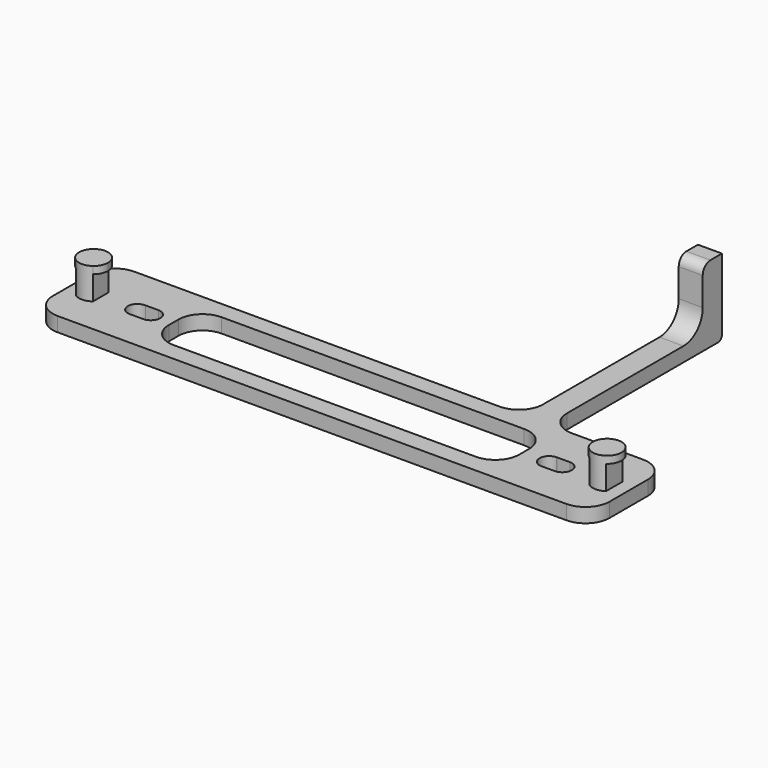
from build123d import *

# Parameters (mm, degrees)
F0_W     = 5
F0_H     = 40.3502766341
F0_H_2   = 5
F0_H_3   = 3.6678295396
F1_DEPTH = 3
F2_DEPTH = 8
F3_START = 8
F3_DEPTH = 1.5
F4_DEPTH = 15.9
F5_R     = 5
F6_R     = 2
F7_R     = 5
F8_R     = 5
F9_R     = 1


# Not quite as in the source:
# - a feature names something its author has since deleted; it is built from what else it names


with BuildPart() as f1:
    # F0 (on Top) → F1 (new body)
    with BuildSketch(Plane.XY):
        Polygon((28.0917086639, 10.1497233659), (-58.0486447513, 10.1497233659), (-58.0486447513, -9.8502766341), (57.9513552487, -9.8502766341), (57.9513552487, 10.1497233659), (33.0917086639, 10.1497233659), (33.0917086639, 6.4818938263), (36.1140687019, 6.4818938263), (36.1140687019, -6.0621835291), (-36.915011704, -6.0621835291), (-36.915011704, 6.4818938263), (28.0917086639, 6.4818938263), align=None)
        with BuildLine():
            ThreePointArc((-51.749339269, 2.5502440972), (-50.8655573089, 1.4917523434), (-50.5486447513, 0.1497233659))
            ThreePointArc((-50.5486447513, 0.1497233659), (-50.8655573089, -1.1923056116), (-51.749339269, -2.2507973654))
            ThreePointArc((-51.749339269, -2.2507973654), (-53.4879347075, -2.8496622863), (-55.249339269, -2.3216402572))
            ThreePointArc((-55.249339269, -2.3216402572), (-56.5486447513, 0.1497233659), (-55.249339269, 2.621086989))
            ThreePointArc((-55.249339269, 2.621086989), (-53.4879347075, 3.1491090181), (-51.749339269, 2.5502440972))
        make_face(mode=Mode.SUBTRACT)
        with BuildLine():
            ThreePointArc((-44.4575695538, -1.9931100518), (-46.2885460051, 0.1122973538), (-44.233055807, 1.9991399955))
            Line((-44.233055807, 1.9991399955), (-41.5036168453, 1.9999999007))
            ThreePointArc((-41.5036168453, 1.9999999007), (-40.0889959767, 1.4144363176), (-39.5029867487, 0))
            ThreePointArc((-39.5029867487, 0), (-40.090424389, -1.4158628395), (-41.5076543288, -1.9999945534))
            Line((-41.5076543288, -1.9999945534), (-44.1351375643, -1.9938625424))
            ThreePointArc((-44.1351375643, -1.9938625424), (-44.296368748, -1.9999945534), (-44.4575695538, -1.9931100518))
        make_face(mode=Mode.SUBTRACT)
        with BuildLine():
            ThreePointArc((44.2317598479, 1.9999996372), (45.6467520995, 1.4146394126), (46.2329645157, 0))
            ThreePointArc((46.2329645157, 0), (45.6471198627, -1.4142717753), (44.2327998612, -1.9999999932))
            Line((44.2327998612, -1.9999999932), (41.528318721, -1.9997773407))
            ThreePointArc((41.528318721, -1.9997773407), (39.4992630702, -0.0561038438), (41.4161207108, 1.998303682))
            ThreePointArc((41.4161207108, 1.998303682), (41.4972713372, 1.9999996372), (41.5784239479, 1.9984014428))
            Line((41.5784239479, 1.9984014428), (44.2317598479, 1.9999996372))
        make_face(mode=Mode.SUBTRACT)
        with BuildLine():
            ThreePointArc((55.1986493307, 2.5883630259), (56.1198644061, 1.5205110508), (56.4513552487, 0.1497233659))
            ThreePointArc((56.4513552487, 0.1497233659), (56.1198644061, -1.221064319), (55.1986493307, -2.288916294))
            ThreePointArc((55.1986493307, -2.288916294), (53.4480237917, -2.8502747843), (51.6986493307, -2.2850295918))
            ThreePointArc((51.6986493307, -2.2850295918), (50.4513552487, 0.1497233659), (51.6986493307, 2.5844763236))
            ThreePointArc((51.6986493307, 2.5844763236), (53.4480237917, 3.1497215161), (55.1986493307, 2.5883630259))
        make_face(mode=Mode.SUBTRACT)
        with BuildLine():
            Line((-51.749339269, 1.7544291914), (-51.749339269, 2.5502440972))
            ThreePointArc((-51.749339269, 2.5502440972), (-53.4879347075, 3.1491090181), (-55.249339269, 2.621086989))
            Line((-55.249339269, 2.621086989), (-55.249339269, 1.7544291914))
            Line((-55.249339269, 1.7544291914), (-51.749339269, 1.7544291914))
        make_face()
        with BuildLine():
            Line((-55.249339269, 1.7544291914), (-55.249339269, 2.621086989))
            ThreePointArc((-55.249339269, 2.621086989), (-56.5486447513, 0.1497233659), (-55.249339269, -2.3216402572))
            Line((-55.249339269, -2.3216402572), (-55.249339269, 1.7544291914))
        make_face()
        with BuildLine():
            ThreePointArc((-55.249339269, -2.3216402572), (-53.4879347075, -2.8496622863), (-51.749339269, -2.2507973654))
            Line((-51.749339269, -2.2507973654), (-51.749339269, 1.7544291914))
            Line((-51.749339269, 1.7544291914), (-55.249339269, 1.7544291914))
            Line((-55.249339269, 1.7544291914), (-55.249339269, -2.3216402572))
        make_face()
        with BuildLine():
            ThreePointArc((-51.749339269, -2.2507973654), (-50.8655573089, -1.1923056116), (-50.5486447513, 0.1497233659))
            ThreePointArc((-50.5486447513, 0.1497233659), (-50.8655573089, 1.4917523434), (-51.749339269, 2.5502440972))
            Line((-51.749339269, 2.5502440972), (-51.749339269, 1.7544291914))
            Line((-51.749339269, 1.7544291914), (-51.749339269, -2.2507973654))
        make_face()
        with BuildLine():
            Line((55.1986493307, 1.9077386241), (55.1986493307, 2.5883630259))
            ThreePointArc((55.1986493307, 2.5883630259), (53.4480237917, 3.1497215161), (51.6986493307, 2.5844763236))
            Line((51.6986493307, 2.5844763236), (51.6986493307, 1.9077386241))
            Line((51.6986493307, 1.9077386241), (55.1986493307, 1.9077386241))
        make_face()
        with BuildLine():
            Line((51.6986493307, 1.9077386241), (51.6986493307, 2.5844763236))
            ThreePointArc((51.6986493307, 2.5844763236), (50.4513552487, 0.1497233659), (51.6986493307, -2.2850295918))
            Line((51.6986493307, -2.2850295918), (51.6986493307, 1.9077386241))
        make_face()
        with BuildLine():
            ThreePointArc((51.6986493307, -2.2850295918), (53.4480237917, -2.8502747843), (55.1986493307, -2.288916294))
            Line((55.1986493307, -2.288916294), (55.1986493307, 1.9077386241))
            Line((55.1986493307, 1.9077386241), (51.6986493307, 1.9077386241))
            Line((51.6986493307, 1.9077386241), (51.6986493307, -2.2850295918))
        make_face()
        with BuildLine():
            ThreePointArc((55.1986493307, -2.288916294), (56.1198644061, -1.221064319), (56.4513552487, 0.1497233659))
            ThreePointArc((56.4513552487, 0.1497233659), (56.1198644061, 1.5205110508), (55.1986493307, 2.5883630259))
            Line((55.1986493307, 2.5883630259), (55.1986493307, 1.9077386241))
            Line((55.1986493307, 1.9077386241), (55.1986493307, -2.288916294))
        make_face()
        with Locations((30.5917086639, 30.324861683)):
            Rectangle(F0_W, F0_H)
        with Locations((30.5917086639, 53)):
            Rectangle(F0_W, F0_H_2)
        with Locations((30.5917086639, 8.3158085961)):
            Rectangle(F0_W, F0_H_3)
    extrude(amount=F1_DEPTH)

    # F0 (on Top) → F2 (join)
    with BuildSketch(Plane.XY):
        with BuildLine():
            ThreePointArc((51.6986493307, -2.2850295918), (53.4480237917, -2.8502747843), (55.1986493307, -2.288916294))
            Line((55.1986493307, -2.288916294), (55.1986493307, 1.9077386241))
            Line((55.1986493307, 1.9077386241), (51.6986493307, 1.9077386241))
            Line((51.6986493307, 1.9077386241), (51.6986493307, -2.2850295918))
        make_face()
        with BuildLine():
            ThreePointArc((-55.249339269, -2.3216402572), (-53.4879347075, -2.8496622863), (-51.749339269, -2.2507973654))
            Line((-51.749339269, -2.2507973654), (-51.749339269, 1.7544291914))
            Line((-51.749339269, 1.7544291914), (-55.249339269, 1.7544291914))
            Line((-55.249339269, 1.7544291914), (-55.249339269, -2.3216402572))
        make_face()
    extrude(amount=F2_DEPTH)

    # F0 (on Top) → F3 (join)
    with BuildSketch(Plane.XY.offset(F3_START)):
        with BuildLine():
            Line((-55.249339269, 1.7544291914), (-55.249339269, 2.621086989))
            ThreePointArc((-55.249339269, 2.621086989), (-56.5486447513, 0.1497233659), (-55.249339269, -2.3216402572))
            Line((-55.249339269, -2.3216402572), (-55.249339269, 1.7544291914))
        make_face()
        with BuildLine():
            Line((-51.749339269, 1.7544291914), (-51.749339269, 2.5502440972))
            ThreePointArc((-51.749339269, 2.5502440972), (-53.4879347075, 3.1491090181), (-55.249339269, 2.621086989))
            Line((-55.249339269, 2.621086989), (-55.249339269, 1.7544291914))
            Line((-55.249339269, 1.7544291914), (-51.749339269, 1.7544291914))
        make_face()
        with BuildLine():
            ThreePointArc((-55.249339269, -2.3216402572), (-53.4879347075, -2.8496622863), (-51.749339269, -2.2507973654))
            Line((-51.749339269, -2.2507973654), (-51.749339269, 1.7544291914))
            Line((-51.749339269, 1.7544291914), (-55.249339269, 1.7544291914))
            Line((-55.249339269, 1.7544291914), (-55.249339269, -2.3216402572))
        make_face()
        with BuildLine():
            ThreePointArc((-51.749339269, -2.2507973654), (-50.8655573089, -1.1923056116), (-50.5486447513, 0.1497233659))
            ThreePointArc((-50.5486447513, 0.1497233659), (-50.8655573089, 1.4917523434), (-51.749339269, 2.5502440972))
            Line((-51.749339269, 2.5502440972), (-51.749339269, 1.7544291914))
            Line((-51.749339269, 1.7544291914), (-51.749339269, -2.2507973654))
        make_face()
        with BuildLine():
            Line((51.6986493307, 1.9077386241), (51.6986493307, 2.5844763236))
            ThreePointArc((51.6986493307, 2.5844763236), (50.4513552487, 0.1497233659), (51.6986493307, -2.2850295918))
            Line((51.6986493307, -2.2850295918), (51.6986493307, 1.9077386241))
        make_face()
        with BuildLine():
            Line((55.1986493307, 1.9077386241), (55.1986493307, 2.5883630259))
            ThreePointArc((55.1986493307, 2.5883630259), (53.4480237917, 3.1497215161), (51.6986493307, 2.5844763236))
            Line((51.6986493307, 2.5844763236), (51.6986493307, 1.9077386241))
            Line((51.6986493307, 1.9077386241), (55.1986493307, 1.9077386241))
        make_face()
        with BuildLine():
            ThreePointArc((51.6986493307, -2.2850295918), (53.4480237917, -2.8502747843), (55.1986493307, -2.288916294))
            Line((55.1986493307, -2.288916294), (55.1986493307, 1.9077386241))
            Line((55.1986493307, 1.9077386241), (51.6986493307, 1.9077386241))
            Line((51.6986493307, 1.9077386241), (51.6986493307, -2.2850295918))
        make_face()
        with BuildLine():
            ThreePointArc((55.1986493307, -2.288916294), (56.1198644061, -1.221064319), (56.4513552487, 0.1497233659))
            ThreePointArc((56.4513552487, 0.1497233659), (56.1198644061, 1.5205110508), (55.1986493307, 2.5883630259))
            Line((55.1986493307, 2.5883630259), (55.1986493307, 1.9077386241))
            Line((55.1986493307, 1.9077386241), (55.1986493307, -2.288916294))
        make_face()
    extrude(amount=F3_DEPTH)

    # F0 (on Top) → F4 (join)
    with BuildSketch(Plane.XY):
        with Locations((30.5917086639, 53)):
            Rectangle(F0_W, F0_H_2)
    extrude(amount=F4_DEPTH)

    # F5
    f5_edges = [f1.edges().sort_by_distance(p)[0] for p in [
        (-58.048645, -9.850277, 1.5),
        (57.951355, -9.850277, 1.5),
        (57.951355, 10.149723, 1.5),
        (-58.048645, 10.149723, 1.5),
    ]]
    fillet(f5_edges, radius=F5_R)

    # F6
    f6_edges = [f1.edges().sort_by_distance(p)[0] for p in [
        (30.591709, 50.5, 15.9),
    ]]
    fillet(f6_edges, radius=F6_R)

    # F7
    f7_edges = [f1.edges().sort_by_distance(p)[0] for p in [
        (-36.915012, 6.481894, 1.5),
        (-36.915012, -6.062184, 1.5),
        (36.114069, -6.062184, 1.5),
        (36.114069, 6.481894, 1.5),
        (28.091709, 10.149723, 1.5),
        (33.091709, 10.149723, 1.5),
    ]]
    fillet(f7_edges, radius=F7_R)

    # F8
    f8_edges = [f1.edges().sort_by_distance(p)[0] for p in [
        (30.591709, 50.5, 3),
    ]]
    fillet(f8_edges, radius=F8_R)

    # F9
    f9_edges = [f1.edges().sort_by_distance(p)[0] for p in [
        (30.591709, 55.5, 0),
    ]]
    fillet(f9_edges, radius=F9_R)


solid = f1.part
